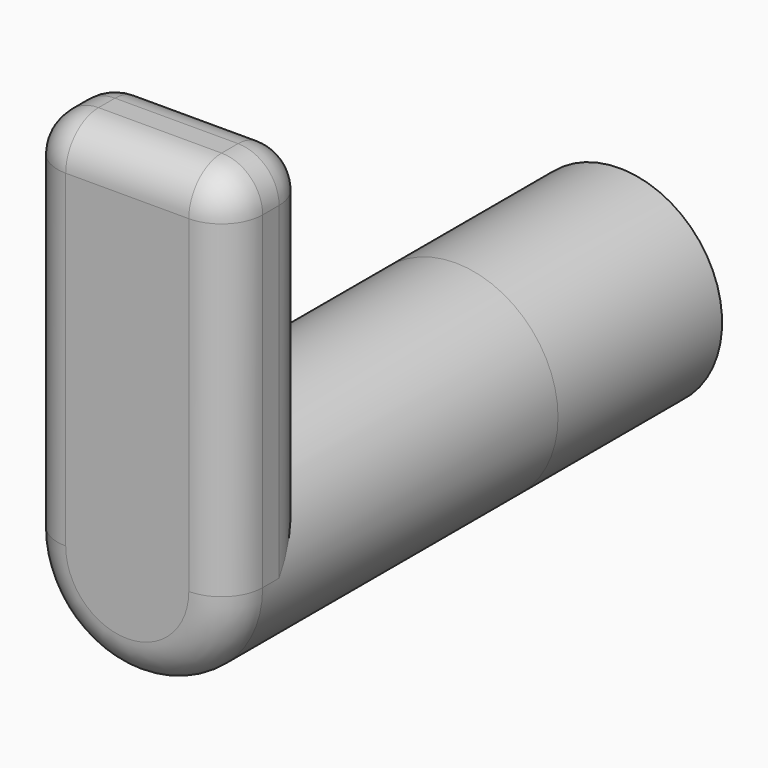
from build123d import *

# Parameters (mm, degrees)
F0_R         = 12.7
F1_DEPTH     = 25.4
F2_W         = 25.4
F2_H         = 12.7
F3_DEPTH     = 45.72
F4_R         = 5.08
F5_T1_DEPTH  = 15.24
F5_T6_DEPTH  = 53.34
F5_S7_R      = 12.7
F5_T8_DEPTH  = 28
F5_T10_ANGLE = 90
F5_T14_DEPTH = 53.34
F5_S15_R     = 12.7
F5_T16_DEPTH = 28
F5_T18_ANGLE = 90
F6_R         = 12.7
F7_DEPTH     = 25.4


# Not quite as in the source:
# - a fillet or chamfer that OpenCascade refuses, or shapes differently, is made with other operations: its cross-section is extruded or revolved along the edge and cut away or added


with BuildPart() as f1:
    # F0 (on Front) → F1 (new body, symmetric)
    with BuildSketch(Plane.XZ):
        Circle(F0_R)
    extrude(amount=F1_DEPTH, both=True)

    # F2 (on Top) → F3 (join)
    with BuildSketch(Plane.XY):
        with Locations((0, -19.05)):
            Rectangle(F2_W, F2_H)
    extrude(amount=F3_DEPTH)

    # F4
    f4_edges = [f1.edges().sort_by_distance(p)[0] for p in [
        (-12.7, -19.05, 45.72),
        (12.7, -19.05, 45.72),
        (0, -25.4, -12.7),
        (0, -25.4, 45.72),
    ]]
    fillet(f4_edges, radius=F4_R)

    # F5: fillet of radius 5.08 on 5 edges, made by hand

    # F5_s2 → F5_t1 (cut)
    with BuildSketch(Plane.YZ.offset(-7.62)):
        with BuildLine():
            ThreePointArc((-12.7, 40.64), (-14.1878975516, 44.2321024484), (-17.78, 45.72))
            Line((-17.78, 45.72), (-12.7, 45.72))
            Line((-12.7, 45.72), (-12.7, 40.64))
        make_face()
    extrude(amount=F5_T1_DEPTH, mode=Mode.SUBTRACT)


with BuildPart() as f5_tool4:
    # F5_s5 → F5_t6 (new body)
    with BuildSketch(Plane.XY.offset(-12.7)):
        with BuildLine():
            ThreePointArc((-12.7, -17.78), (-11.2121024484, -14.1878975516), (-7.62, -12.7))
            Line((-7.62, -12.7), (-12.7, -12.7))
            Line((-12.7, -12.7), (-12.7, -17.78))
        make_face()
    extrude(amount=F5_T6_DEPTH)

    # F5_s7 → F5_t8 (cut, symmetric)
    with BuildSketch(Plane.XZ.offset(15.2)):
        Circle(F5_S7_R)
    extrude(amount=F5_T8_DEPTH, both=True, mode=Mode.SUBTRACT)


with BuildPart() as f1_1:
    add(f1.part)

    # F5_t3: cut F5_tool4
    add(f5_tool4.part, mode=Mode.SUBTRACT)

    # F5_s9 → F5_t10 (revolve, cut)
    with BuildSketch(Plane.XY.offset(40.64)):
        with BuildLine():
            ThreePointArc((-7.62, -12.7), (-11.2121024484, -14.1878975516), (-12.7, -17.78))
            Line((-12.7, -17.78), (-12.7, -12.7))
            Line((-12.7, -12.7), (-7.62, -12.7))
        make_face()
    revolve(axis=Axis((-7.62, -12.7, 40.64), (0, 1, 0)), revolution_arc=F5_T10_ANGLE, mode=Mode.SUBTRACT)


with BuildPart() as f5_tool12:
    # F5_s13 → F5_t14 (new body)
    with BuildSketch(Plane.XY.offset(-12.7)):
        with BuildLine():
            ThreePointArc((7.62, -12.7), (11.2121024484, -14.1878975516), (12.7, -17.78))
            Line((12.7, -17.78), (12.7, -12.7))
            Line((12.7, -12.7), (7.62, -12.7))
        make_face()
    extrude(amount=F5_T14_DEPTH)

    # F5_s15 → F5_t16 (cut, symmetric)
    with BuildSketch(Plane.XZ.offset(15.2)):
        Circle(F5_S15_R)
    extrude(amount=F5_T16_DEPTH, both=True, mode=Mode.SUBTRACT)


with BuildPart() as f1_2:
    add(f1_1.part)

    # F5_t11: cut F5_tool12
    add(f5_tool12.part, mode=Mode.SUBTRACT)

    # F5_s17 → F5_t18 (revolve, cut)
    with BuildSketch(Plane.XY.offset(40.64)):
        with BuildLine():
            ThreePointArc((7.62, -12.7), (11.2121024484, -14.1878975516), (12.7, -17.78))
            Line((12.7, -17.78), (12.7, -12.7))
            Line((12.7, -12.7), (7.62, -12.7))
        make_face()
    revolve(axis=Axis((7.62, -12.7, 40.64), (0, -1, 0)), revolution_arc=F5_T18_ANGLE, mode=Mode.SUBTRACT)

    # F6 (on face) → F7 (join)
    with BuildSketch(Plane(origin=(0, 25.4, 0), x_dir=(-1, 0, 0), z_dir=(0, 1, 0))):
        Circle(F6_R)
    extrude(amount=F7_DEPTH)


solid = f1_2.part
